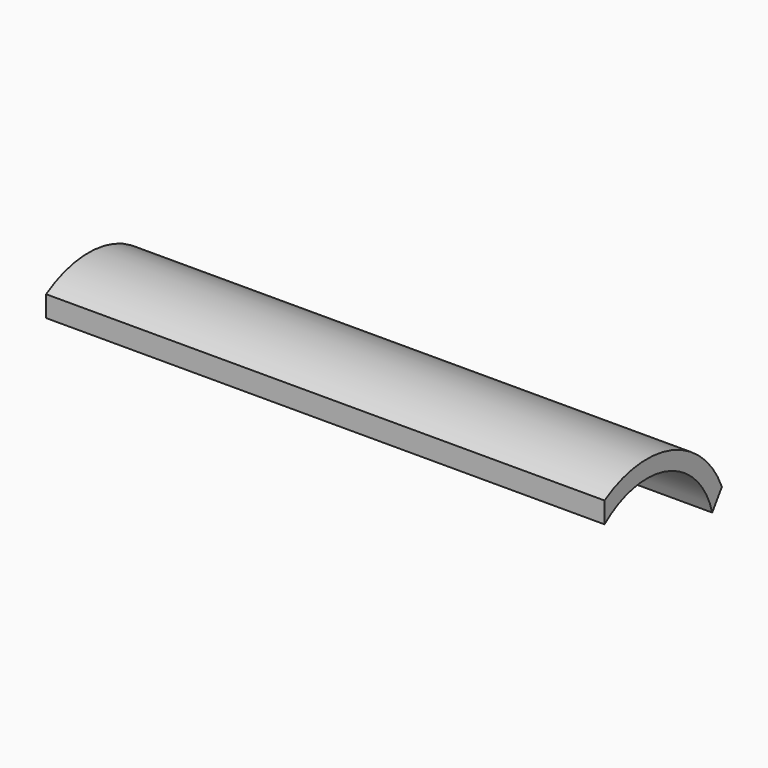
from build123d import *


# Not quite as in the source:
# - a feature names something its author has since deleted; it is built from what else it names


with BuildPart() as f2:
    # F2: sweep along a path in F0
    with BuildLine(Plane.XZ) as f2_path:
        Line((-25.6183743477, 3.866331419), (-7.8389644623, 3.866331419))
    # F1 (on Right) → F2 (sweep)
    with BuildSketch(Plane.YZ):
        with BuildLine():
            Line((1.5781502627, 3.0087089686), (1.9656477529, 3.5727088214))
            ThreePointArc((1.9656477529, 3.5727088214), (-0.020304079, 5.4099020075), (-2.7067011688, 5.0896612265))
            Line((-2.7067011688, 5.0896612265), (-2.7067011688, 4.4201179408))
            ThreePointArc((-2.7067011688, 4.4201179408), (-0.1784378749, 4.8857654381), (1.5781502627, 3.0087089686))
        make_face()
    sweep(path=f2_path.line)


solid = f2.part
